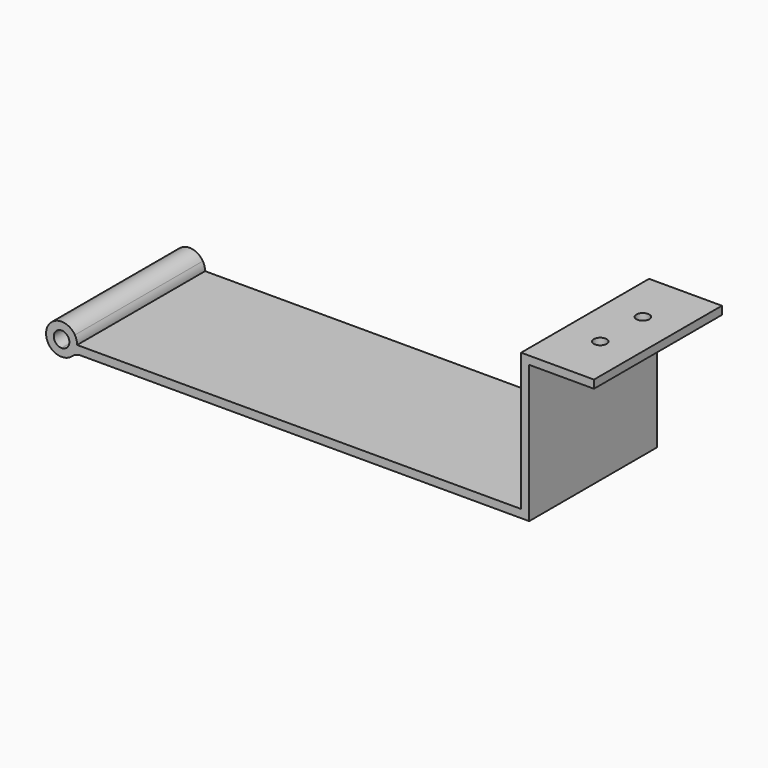
from build123d import *

# Parameters (mm, degrees)
F0_W     = 3.175
F0_H     = 3.175
F0_W_2   = 25.4
F1_DEPTH = 62.7250036666
F2_R     = 5.08
F3_R     = 2.54
F4_DEPTH = 60.072


with BuildPart() as f1:
    # F0 (on Front) → F1 (new body)
    with BuildSketch(Plane.XZ):
        with BuildLine():
            Line((-47.2060584766, 11.2612042576), (-47.2060584766, 14.4362042576))
            ThreePointArc((-47.2060584766, 14.4362042576), (-47.4333192743, 12.7872299777), (-48.0981569595, 11.2612042576))
            Line((-48.0981569595, 11.2612042576), (-47.2060584766, 11.2612042576))
        make_face()
        Polygon((126.9109415234, 14.4362042576), (-47.2060584766, 14.4362042576), (-47.2060584766, 11.2612042576), (130.0859415234, 11.2612042576), (130.0859415234, 14.4362042576), align=None)
        with BuildLine():
            ThreePointArc((-48.0981569595, 11.2612042576), (-47.4333192743, 12.7872299777), (-47.2060584766, 14.4362042576))
            ThreePointArc((-47.2060584766, 14.4362042576), (-47.4333192743, 16.0851785375), (-48.0981569595, 17.6112042576))
            ThreePointArc((-48.0981569595, 17.6112042576), (-53.3020584766, 20.5322042576), (-58.5059599937, 17.6112042576))
            ThreePointArc((-58.5059599937, 17.6112042576), (-59.3980584766, 14.4362042576), (-58.5059599937, 11.2612042576))
            ThreePointArc((-58.5059599937, 11.2612042576), (-53.3020584766, 8.3402042576), (-48.0981569595, 11.2612042576))
        make_face()
        with BuildLine():
            ThreePointArc((-53.3020584766, 17.4842042576), (-51.1467970075, 16.5914657267), (-50.2540584766, 14.4362042576))
            ThreePointArc((-50.2540584766, 14.4362042576), (-51.1467970075, 12.2809427886), (-53.3020584766, 11.3882042576))
            ThreePointArc((-53.3020584766, 11.3882042576), (-56.3500584766, 14.4362042576), (-53.3020584766, 17.4842042576))
        make_face(mode=Mode.SUBTRACT)
        Polygon((126.9109415234, 68.4112042576), (126.9109415234, 17.6112042576), (130.0859415234, 17.6112042576), (130.0859415234, 65.2362042576), (130.0859415234, 68.4112042576), align=None)
        with Locations((128.4984415234, 16.0237042576)):
            Rectangle(F0_W, F0_H)
        with Locations((142.7859415234, 66.8237042576)):
            Rectangle(F0_W_2, F0_H)
    extrude(amount=F1_DEPTH)

    # F2
    f2_edges = [f1.edges().sort_by_distance(p)[0] for p in [
        (-48.098157, -31.362502, 11.261204),
    ]]
    fillet(f2_edges, radius=F2_R)

    # F3 (on face) → F4 (cut, through all)
    with BuildSketch(Plane.XY.offset(68.4112042576)):
        with Locations((141.1984415234, -20.9083345554)):
            Circle(F3_R)
        with Locations((141.1984415234, -41.8166691112)):
            Circle(F3_R)
    extrude(amount=-F4_DEPTH, mode=Mode.SUBTRACT)


solid = f1.part
